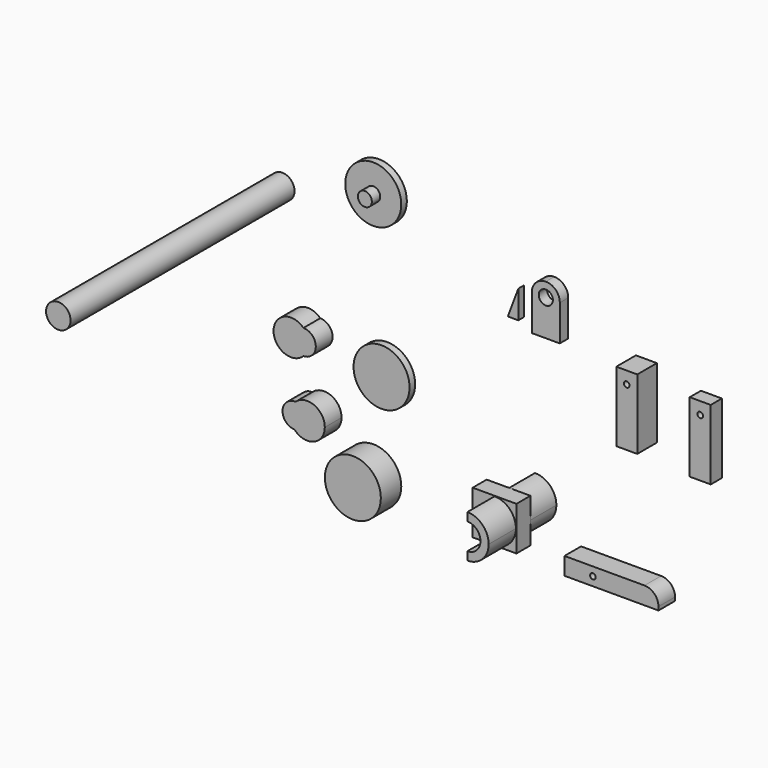
from build123d import *

# Parameters (mm, degrees)
F0_W           = 15.875
F0_H           = 15.875
F1_DEPTH       = 6.35
F0_W_2         = 34.115
F0_H_2         = 6.35
F0_R           = 1.016
F2_DEPTH       = 7.52
F3_DEPTH       = 7.62
F0_R_2         = 10.16
F4_DEPTH       = 9.271
F5_R           = 5.08
F6_DEPTH       = 2.54
F0_R_3         = 2.54
F7_DEPTH       = 6.35
F8_DEPTH       = 2.54
F9_DEPTH       = 3.81
F10_DEPTH      = 2.54
F11_R          = 5.07999
F12_DEPTH      = 7.62
F13_DEPTH      = 5.08
F14_DEPTH      = 8.9
F0_R_4         = 4.445
F15_DEPTH      = 101.6
F16_DEPTH      = 6.35
F17_DEPTH      = 18.7
F17_DEPTH_BACK = 12


# Not quite as in the source:
# - a fillet or chamfer is up to 0.001 mm smaller than in the source, because OpenCascade refuses the exact size
# - a length typed as a fraction of an inch, garbled in the dataset ("3 / 203.2 mm" for 3/8 in), is restored


with BuildPart() as f1:
    # F0 (on Front) → F1 (new body)
    with BuildSketch(Plane.XZ):
        with Locations((13.4390089661, -39.8432931602)):
            Rectangle(F0_W, F0_H)
        with BuildLine():
            ThreePointArc((13.4390089661, -47.5932931602), (5.6890089661, -39.8432931602), (13.4390089661, -32.0932931602))
            ThreePointArc((13.4390089661, -32.0932931602), (18.9190865203, -34.363215606), (21.1890089661, -39.8432931602))
            ThreePointArc((21.1890089661, -39.8432931602), (18.9190865203, -45.3233707144), (13.4390089661, -47.5932931602))
        make_face(mode=Mode.SUBTRACT)
    extrude(amount=F1_DEPTH)

    # F0 (on Front) → F16 (join)
    with BuildSketch(Plane.XZ):
        with BuildLine():
            ThreePointArc((13.4390089661, -44.6057931602), (8.6765089661, -39.8432931602), (13.4390089661, -35.0807931602))
            Line((13.4390089661, -35.0807931602), (13.4390089661, -32.0932931602))
            ThreePointArc((13.4390089661, -32.0932931602), (5.6890089661, -39.8432931602), (13.4390089661, -47.5932931602))
            Line((13.4390089661, -47.5932931602), (13.4390089661, -44.6057931602))
        make_face()
    extrude(amount=F16_DEPTH)

    # F0 (on Front) → F17 (join, two sides)
    with BuildSketch(Plane.XZ) as f17_sk:
        with BuildLine():
            ThreePointArc((13.4390089661, -35.0807931602), (16.8066050115, -36.4756971148), (18.2015089661, -39.8432931602))
            ThreePointArc((18.2015089661, -39.8432931602), (16.8066050115, -43.2108892056), (13.4390089661, -44.6057931602))
            Line((13.4390089661, -44.6057931602), (13.4390089661, -47.5932931602))
            ThreePointArc((13.4390089661, -47.5932931602), (18.9190865203, -45.3233707144), (21.1890089661, -39.8432931602))
            ThreePointArc((21.1890089661, -39.8432931602), (18.9190865203, -34.363215606), (13.4390089661, -32.0932931602))
            Line((13.4390089661, -32.0932931602), (13.4390089661, -35.0807931602))
        make_face()
    extrude(amount=F17_DEPTH)
    extrude(f17_sk.sketch, amount=-F17_DEPTH_BACK)


with BuildPart() as f2:
    # F0 (on Front) → F2 (new body)
    with BuildSketch(Plane.XZ):
        with Locations((56.8083405149, -45.2704743564)):
            Rectangle(F0_W_2, F0_H_2)
        with Locations((50.0551967038, -45.2725063564)):
            Circle(F0_R, mode=Mode.SUBTRACT)
    extrude(amount=F2_DEPTH)

    # F5
    f5_edges = [f2.edges().sort_by_distance(p)[0] for p in [
        (73.865841, -3.76, -42.095474),
    ]]
    fillet(f5_edges, radius=F5_R)


with BuildPart() as f3:
    # F0 (on Front) → F3 (new body)
    with BuildSketch(Plane.XZ):
        with BuildLine():
            ThreePointArc((-58.1704086232, -33.5221318855), (-51.1918348413, -35.1302957719), (-47.1535133362, -29.2160212994))
            ThreePointArc((-47.1535133362, -29.2160212994), (-50.9520649509, -23.4011600682), (-57.8031546393, -24.5431651423))
            ThreePointArc((-57.8031546393, -24.5431651423), (-59.8482084076, -28.9565132058), (-58.1704086232, -33.5221318855))
        make_face()
        with BuildLine():
            ThreePointArc((-58.1704086232, -33.5221318855), (-59.8482084076, -28.9565132058), (-57.8031546393, -24.5431651423))
            ThreePointArc((-57.8031546393, -24.5431651423), (-62.483722892, -28.8487164825), (-58.1704086232, -33.5221318855))
        make_face()
    extrude(amount=F3_DEPTH)


with BuildPart() as f4:
    # F0 (on Front) → F4 (new body)
    with BuildSketch(Plane.XZ):
        with Locations((-35.6504768133, -44.1323518753)):
            Circle(F0_R_2)
    extrude(amount=F4_DEPTH)


with BuildPart() as f6:
    # F0 (on Front) → F6 (new body)
    with BuildSketch(Plane.XZ):
        with Locations((-30.6192673743, -9.8629677668)):
            Circle(F0_R_2)
    extrude(amount=F6_DEPTH)


with BuildPart() as f7:
    # F0 (on Front) → F7 (new body)
    with BuildSketch(Plane.XZ):
        with Locations((-33.6301475763, 47.6013273001)):
            Circle(F0_R_3)
    extrude(amount=F7_DEPTH)

    # F0 (on Front) → F8 (join)
    with BuildSketch(Plane.XZ):
        with Locations((-33.6301475763, 47.6013273001)):
            Circle(F0_R_2)
        with Locations((-33.6301475763, 47.6013273001)):
            Circle(F0_R_3, mode=Mode.SUBTRACT)
    extrude(amount=F8_DEPTH)


with BuildPart() as f9:
    # F0 (on Front) → F9 (new body)
    with BuildSketch(Plane.XZ):
        with BuildLine():
            Line((27.4471032315, 35.7939480323), (24.9321032315, 35.7939480323))
            Line((24.9321032315, 35.7939480323), (24.9321032315, 22.7639480323))
            Line((24.9321032315, 22.7639480323), (35.0921032315, 22.7639480323))
            Line((35.0921032315, 22.7639480323), (35.0921032315, 35.7939480323))
            Line((35.0921032315, 35.7939480323), (32.5771032315, 35.7939480323))
            ThreePointArc((32.5771032315, 35.7939480323), (30.0121032315, 33.2289480323), (27.4471032315, 35.7939480323))
        make_face()
        with BuildLine():
            Line((35.0921032315, 40.8739480323), (24.9321032315, 40.8739480323))
            Line((24.9321032315, 40.8739480323), (24.9321032315, 35.7939480323))
            Line((24.9321032315, 35.7939480323), (27.4471032315, 35.7939480323))
            ThreePointArc((27.4471032315, 35.7939480323), (30.0121032315, 38.3589480323), (32.5771032315, 35.7939480323))
            Line((32.5771032315, 35.7939480323), (35.0921032315, 35.7939480323))
            Line((35.0921032315, 35.7939480323), (35.0921032315, 40.8739480323))
        make_face()
    extrude(amount=F9_DEPTH)

    # F11 (radius 5.08 in the source; OpenCascade refuses exactly that, so slightly less here)
    f11_edges = [f9.edges().sort_by_distance(p)[0] for p in [
        (35.092103, -1.905, 40.873948),
        (24.932103, -1.905, 40.873948),
    ]]
    fillet(f11_edges, radius=F11_R)


with BuildPart() as f10:
    # F0 (on Front) → F10 (new body)
    with BuildSketch(Plane.XZ):
        Polygon((19.0205297893, 24.3973601609), (19.0205297893, 34.5573601609), (15.2105297893, 24.3973601609), align=None)
    extrude(amount=F10_DEPTH)


with BuildPart() as f12:
    # F0 (on Front) → F12 (new body)
    with BuildSketch(Plane.XZ):
        with BuildLine():
            ThreePointArc((-54.9034981155, -8.9814396879), (-53.5265594418, -6.9211462608), (-53.0430343145, -4.490719844))
            ThreePointArc((-53.0430343145, -4.490719844), (-53.5265594418, -2.0602934271), (-54.9034981155, 0))
            ThreePointArc((-54.9034981155, 0), (-65.7430343145, -4.490719844), (-54.9034981155, -8.9814396879))
        make_face()
        with BuildLine():
            ThreePointArc((-54.9034981155, 0), (-53.5265594418, -2.0602934271), (-53.0430343145, -4.490719844))
            ThreePointArc((-53.0430343145, -4.490719844), (-53.5265594418, -6.9211462608), (-54.9034981155, -8.9814396879))
            ThreePointArc((-54.9034981155, -8.9814396879), (-50.4115943145, -4.490719844), (-54.9034981155, 0))
        make_face()
    extrude(amount=F12_DEPTH)


with BuildPart() as f13:
    # F0 (on Front) → F13 (new body)
    with BuildSketch(Plane.XZ):
        with BuildLine():
            Line((90.8731772517, 21.7727785543), (83.2531772517, 21.7727785543))
            Line((83.2531772517, 21.7727785543), (83.2531772517, 17.3277785543))
            Line((83.2531772517, 17.3277785543), (86.0471772517, 17.3277785543))
            ThreePointArc((86.0471772517, 17.3277785543), (87.0631772517, 18.3437785543), (88.0791772517, 17.3277785543))
            Line((88.0791772517, 17.3277785543), (90.8731772517, 17.3277785543))
            Line((90.8731772517, 17.3277785543), (90.8731772517, 21.7727785543))
        make_face()
        with BuildLine():
            Line((86.0471772517, 17.3277785543), (83.2531772517, 17.3277785543))
            Line((83.2531772517, 17.3277785543), (83.2531772517, -3.6272214457))
            Line((83.2531772517, -3.6272214457), (90.8731772517, -3.6272214457))
            Line((90.8731772517, -3.6272214457), (90.8731772517, 17.3277785543))
            Line((90.8731772517, 17.3277785543), (88.0791772517, 17.3277785543))
            ThreePointArc((88.0791772517, 17.3277785543), (87.0631772517, 16.3117785543), (86.0471772517, 17.3277785543))
        make_face()
    extrude(amount=F13_DEPTH)


with BuildPart() as f14:
    # F0 (on Front) → F14 (new body)
    with BuildSketch(Plane.XZ):
        with BuildLine():
            Line((67.2715870141, 25.4), (59.6515870141, 25.4))
            Line((59.6515870141, 25.4), (59.6515870141, 21.2394388122))
            Line((59.6515870141, 21.2394388122), (62.4663369513, 21.2394388122))
            ThreePointArc((62.4663369513, 21.2394388122), (63.5645068324, 21.9635517753), (64.456837077, 20.9970822176))
            Line((64.456837077, 20.9970822176), (67.2715870141, 20.9970822176))
            Line((67.2715870141, 20.9970822176), (67.2715870141, 25.4))
        make_face()
        with BuildLine():
            Line((62.4663369513, 21.2394388122), (59.6515870141, 21.2394388122))
            Line((59.6515870141, 21.2394388122), (59.6515870141, 0))
            Line((59.6515870141, 0), (67.2715870141, 0))
            Line((67.2715870141, 0), (67.2715870141, 20.9970822176))
            Line((67.2715870141, 20.9970822176), (64.456837077, 20.9970822176))
            ThreePointArc((64.456837077, 20.9970822176), (64.4574909684, 20.9760456244), (64.4577089634, 20.955))
            ThreePointArc((64.4577089634, 20.955), (63.2980461018, 19.9492082809), (62.4663369513, 21.2394388122))
        make_face()
    extrude(amount=F14_DEPTH)


with BuildPart() as f15:
    # F0 (on Front) → F15 (new body)
    with BuildSketch(Plane.XZ):
        with Locations((-68.6774551868, 37.5820547342)):
            Circle(F0_R_4)
    extrude(amount=F15_DEPTH)


solid = Compound([f1.part, f2.part, f3.part, f4.part, f6.part, f7.part, f9.part, f10.part, f12.part, f13.part, f14.part, f15.part])
